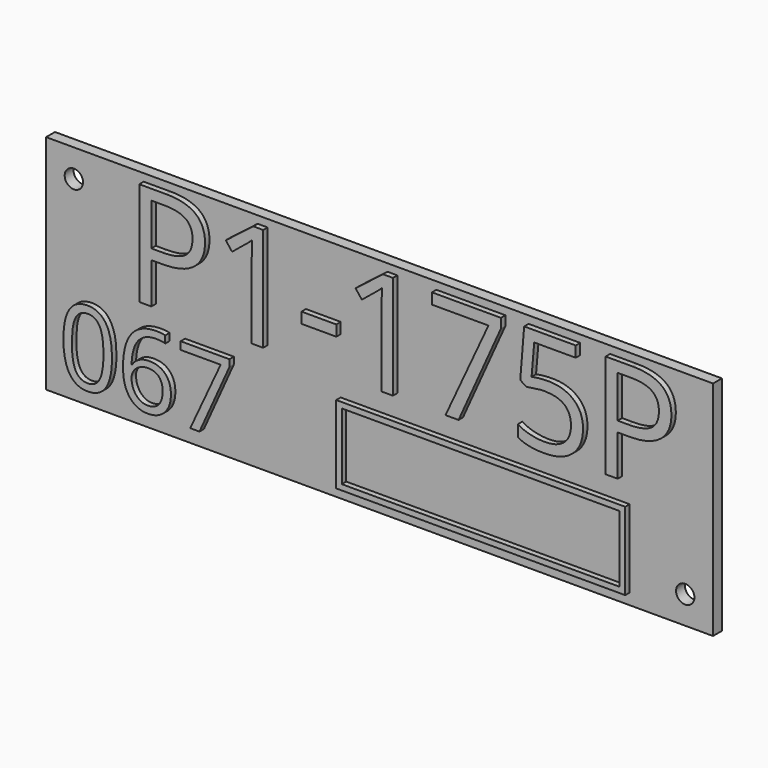
from build123d import *

# Parameters (mm, degrees)
F0_W         = 120
F0_H         = 40
F1_DEPTH     = 2
F3_D         = 3.3
F4_TEXT_SIZE = 26.1352499183
F5_DEPTH     = 1
F6_TEXT_SIZE = 18.5054667028
F7_DEPTH     = 1
F8_W         = 52
F8_H         = 14
F8_W_2       = 49.99999962
F8_H_2       = 11.99999962
F9_DEPTH     = 1


# Not quite as in the source:
# - Text() gives the source's letters only with a copy of the font that has no kerning and outlines rounded to 1/6400 em; it was checked with that copy


with BuildPart() as f1:
    # F0 (on Front) → F1 (new body)
    with BuildSketch(Plane.XZ):
        Rectangle(F0_W, F0_H)
    extrude(amount=F1_DEPTH)

    # F3 (through all)
    with Locations(Plane.XZ.offset(2)):
        with Locations((-55, 15), (55, -15)):
            Hole(F3_D / 2)

    # F4 (on face) → F5 (join)
    with BuildSketch(Plane.XZ.offset(2)):
        with Locations((-45, 0)):
            Text('P1-175P', F4_TEXT_SIZE, font='Open Sans', text_align=(TextAlign.LEFT, TextAlign.BOTTOM))
    extrude(amount=F5_DEPTH)

    # F6 (on face) → F7 (join)
    with BuildSketch(Plane.XZ.offset(2)):
        with Locations((-57, -17)):
            Text('067', F6_TEXT_SIZE, font='Open Sans', text_align=(TextAlign.LEFT, TextAlign.BOTTOM))
    extrude(amount=F7_DEPTH)

    # F8 (on face) → F9 (join)
    with BuildSketch(Plane.XZ.offset(2)):
        with Locations((19, -11)):
            Rectangle(F8_W, F8_H)
        with Locations((19, -11)):
            Rectangle(F8_W_2, F8_H_2, mode=Mode.SUBTRACT)
    extrude(amount=F9_DEPTH)


solid = f1.part
